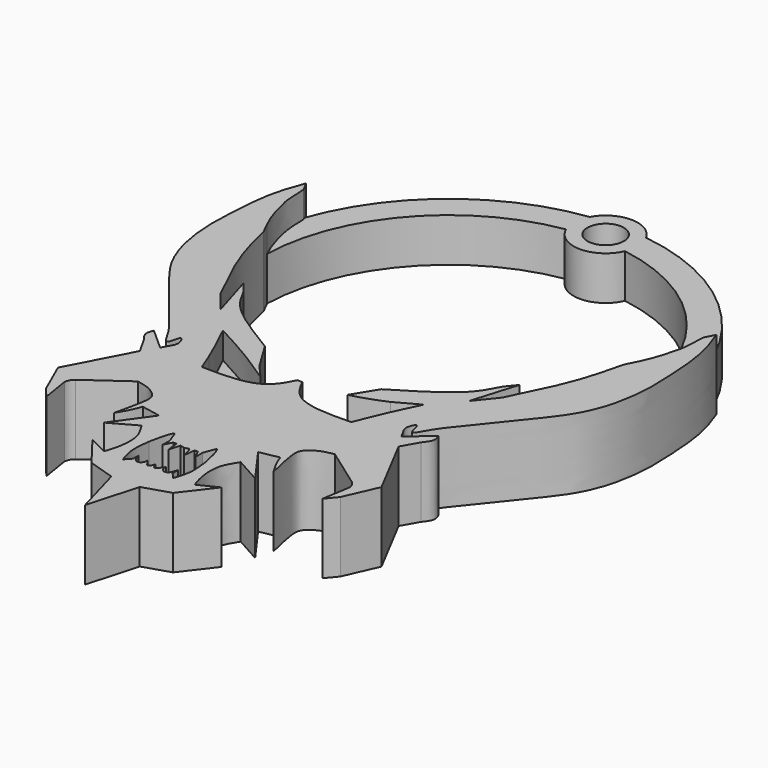
from build123d import *

# Parameters (mm, degrees)
F1_DEPTH = 6.096
F0_R     = 1.5875
F2_DEPTH = 3.81


# Not quite as in the source:
# - a feature names something its author has since deleted; it is built from what else it names


with BuildPart() as f1:
    # F0 (on Top) → F1 (new body)
    with BuildSketch(Plane.XY):
        with BuildLine():
            add(Edge.make_bspline(
                [(0.5293725099, -15.6763419509), (0.5292411185, -15.0751519368), (0.5291231168, -14.1058757461), (-0.304833504, -14.3066064417), (-0.702635768, -15.0022322051), (-0.8362339781, -15.6491980957), (-0.9058115984, -15.9958619624)],
                knots=[0, 0, 0, 0, 0.3108352553, 0.5010759779, 0.7328053585, 1, 1, 1, 1], degree=3))
            Line((-0.9058115984, -15.9958619624), (-0.9058115984, -17.2402724717))
            Line((-0.9058115984, -17.2402724717), (-0.9058115984, -20.226017161))
            Line((-0.9058115984, -20.226017161), (-0.4975165666, -20.1146639884))
            Line((-0.4975165666, -20.1146639884), (-0.2333296888, -21.083349362))
            Line((-0.2333296888, -21.083349362), (-0.120106708, -20.0769230723))
            Line((-0.120106708, -20.0769230723), (0.1692407805, -20.0769230723))
            Line((0.1692407805, -20.0769230723), (0.5214897956, -20.7814220339))
            Line((0.5214897956, -20.7814220339), (0.5214897956, -20.0140215456))
            Line((0.5214897956, -20.0140215456), (0.9240602649, -18.9321134239))
            add(Edge.make_bspline(
                [(1.5430712647, -20.99862881), (1.4140985421, -20.3755580817), (1.2139097457, -19.4084405646), (1.0001161662, -19.0571006756), (0.9240602649, -18.9321134239)],
                knots=[0, 0, 0, 0, 0.6442554471, 1, 1, 1, 1], degree=3))
            add(Edge.make_bspline(
                [(1.5430712647, -20.99862881), (1.5891426732, -21.3454236442), (1.6801064412, -22.0301382187), (1.6564477656, -23.027052549), (1.4157694303, -23.7757681603), (1.2894679367, -24.1686739028)],
                knots=[0, 0, 0, 0, 0.3278252251, 0.6472608224, 1, 1, 1, 1], degree=3))
            Line((1.2894679367, -24.1686739028), (0.8139614056, -23.6456152052))
            Line((0.8139614056, -23.6456152052), (0.8139614056, -23.0591576546))
            Line((0.8139614056, -23.0591576546), (0.6237587932, -23.5980655998))
            add(Edge.make_bspline(
                [(0.6237587932, -23.5980655998), (0.5203329412, -23.7070830693), (0.3117783718, -23.9269129374), (-0.1343922109, -23.6183458648), (-0.1149094653, -23.3495364146), (-0.1053512988, -23.2176594436)],
                knots=[0, 0, 0, 0, 0.3338450489, 0.6731867236, 1, 1, 1, 1], degree=3))
            add(Edge.make_bspline(
                [(-0.1053512988, -23.2176594436), (-0.1910648023, -23.3432038696), (-0.3485399431, -23.5738574464), (-0.6633676878, -23.9588387788), (-0.8187055947, -23.5684484666), (-0.9058115984, -23.3495364146)],
                knots=[0, 0, 0, 0, 0.3441103437, 0.6322087254, 1, 1, 1, 1], degree=3))
            Line((-0.9058115984, -23.3495364146), (-0.9058115984, -31.032309746))
            Line((-0.9058115984, -31.032309746), (0.3292436286, -26.6169421375))
            Line((0.3292436286, -26.6169421375), (2.6450775604, -25.8826520294))
            Line((2.6450775604, -25.8826520294), (4.7067347023, -23.1996756047))
            Line((4.7067347023, -23.1996756047), (3.0404640402, -24.01868999))
            add(Edge.make_bspline(
                [(3.4076086286, -19.4717478007), (3.0937385558, -19.9567840389), (2.4453216005, -20.9588092337), (2.6790373281, -23.0215383373), (2.9334509144, -23.7234480732), (3.0404640402, -24.01868999)],
                knots=[0, 0, 0, 0, 0.352149071, 0.7274966562, 1, 1, 1, 1], degree=3))
            Line((3.4076086286, -19.4717478007), (5.6746407577, -20.7343993974))
            Line((5.6746407577, -20.7343993974), (3.4076086286, -17.5788570195))
            Line((3.4076086286, -17.5788570195), (5.0825377966, -17.2539744526))
            add(Edge.make_bspline(
                [(5.0825377966, -17.2539744526), (4.8011213396, -16.399087297), (4.561581244, -14.6768120309), (3.8789077119, -13.3473311872), (2.9929043757, -14.0969088604), (2.5971549398, -15.3576013762), (2.3466445546, -16.1556228995)],
                knots=[0.2245927854, 0.2245927854, 0.2245927854, 0.2245927854, 0.4782852707, 0.6388064134, 0.7713635541, 1, 1, 1, 1], degree=3))
            add(Edge.make_bspline(
                [(2.3466445546, -16.1556228995), (2.3842676065, -15.6562172431), (2.446566596, -14.829264983), (2.0863685782, -14.1048130028), (1.1405428731, -14.5139735511), (0.7504573644, -15.2558666398), (0.5293725099, -15.6763419509)],
                knots=[0, 0, 0, 0, 0.293818077, 0.4865253721, 0.7089831309, 1, 1, 1, 1], degree=3))
        make_face()
        with BuildLine():
            add(Edge.make_bspline(
                [(-2.3409957066, -15.6763419509), (-2.3408643153, -15.0751519368), (-2.3407463136, -14.1058757461), (-1.5067896928, -14.3066064417), (-1.1089874287, -15.0022322051), (-0.9753892187, -15.6491980957), (-0.9058115984, -15.9958619624)],
                knots=[0, 0, 0, 0, 0.3108352553, 0.5010759779, 0.7328053585, 1, 1, 1, 1], degree=3))
            Line((-0.9058115984, -15.9958619624), (-0.9058115984, -10.0475378801))
            ThreePointArc((-0.9058115984, -10.0475378801), (-2.1470576627, -10.0060667495), (-3.3827675581, -9.8818383259))
            add(Edge.make_bspline(
                [(-7.4073243886, -10.1740490645), (-6.8075722055, -10.1898428856), (-5.6994728773, -10.2190234756), (-4.0527664378, -10.086462301), (-3.3827675581, -9.8818383259)],
                knots=[0, 0, 0, 0, 0.2907722774, 0.5372294996, 0.5372294996, 0.5372294996, 0.5372294996], degree=3))
            add(Edge.make_bspline(
                [(-8.0257326858, -8.6305521925), (-7.8097104935, -9.1525428167), (-7.6085174411, -9.6632959406), (-7.4073243886, -10.1740490645)],
                knots=[0.6828872742, 0.6828872742, 0.6828872742, 0.6828872742, 1, 1, 1, 1], degree=3))
            ThreePointArc((-8.0257326858, -8.6305521925), (-17.8922818311, 0.9803936451), (-18.4399173864, 14.7433572514))
            Line((-18.4399173864, 14.7433572514), (-18.763165921, 15.3649877757))
            add(Edge.make_bspline(
                [(-18.763165921, 15.3649877757), (-19.0883395817, 14.5086239338), (-19.7992570018, 12.636390561), (-20.0614592208, 8.5203671128), (-20.1450147574, 5.8595589947), (-19.6738988858, 2.8012720369), (-18.6296468166, 0.3216380832), (-17.0091341275, -1.7743617945), (-15.3450751303, -3.7604958896), (-13.6655248013, -5.9244622505), (-12.3083012645, -7.5657887279), (-11.4854032906, -9.3943366521), (-11.2878987157, -7.2532302498), (-10.7636393615, -8.3629400774), (-10.8566466443, -8.6570845714), (-10.8958482742, -8.7963175029)],
                knots=[0, 0, 0, 0, 0.0909432234, 0.1983591023, 0.2866981591, 0.3790334905, 0.4664436369, 0.5525333062, 0.6387369107, 0.7267051925, 0.8096970964, 0.865554309, 0.9200718235, 0.9623434622, 1, 1, 1, 1], degree=3))
            Line((-10.8958482742, -8.7963175029), (-11.4042023197, -9.7282994539))
            Line((-11.4042023197, -9.7282994539), (-13.2964076474, -8.0337869003))
            add(Edge.make_bspline(
                [(-13.2964076474, -8.0337869003), (-13.3911344335, -8.2566997732), (-13.5964633769, -8.7398837438), (-13.1995487174, -9.2537872923), (-12.9857473075, -9.5306057483)],
                knots=[0, 0, 0, 0, 0.4613416139, 1, 1, 1, 1], degree=3))
            Line((-12.9857473075, -9.5306057483), (-12.1667329222, -10.9709417447))
            Line((-12.1667329222, -10.9709417447), (-14.9909211323, -16.3651406765))
            Line((-14.9909211323, -16.3651406765), (-13.7200364843, -19.2458126694))
            Line((-13.7200364843, -19.2458126694), (-12.9292635247, -20.2060360461))
            Line((-12.9292635247, -20.2060360461), (-13.3246500045, -17.7489928901))
            add(Edge.make_bspline(
                [(-13.3246500045, -17.7489928901), (-13.3045380935, -17.4936130643), (-13.1847178563, -17.21403189), (-12.9292635247, -17.0147046447)],
                knots=[0, 0, 0, 0, 0.8339722392, 0.8339722392, 0.8339722392, 0.8339722392], degree=3))
            Line((-12.9292635247, -17.0147046447), (-9.4837546349, -14.5576605573))
            add(Edge.make_bspline(
                [(-9.4837546349, -14.5576605573), (-9.1155322754, -14.6255809567), (-8.3698134561, -14.7631324083), (-7.2411030981, -15.5377610794), (-7.2707455103, -16.6588016712), (-7.6292823128, -18.2311499304), (-7.8527219594, -19.2110352218)],
                knots=[0, 0, 0, 0, 0.2233158358, 0.4522561359, 0.6586467707, 1, 1, 1, 1], degree=3))
            add(Edge.make_bspline(
                [(-7.8527219594, -19.2110352218), (-7.4980098211, -18.6109186621), (-7.1432976829, -18.0108021025), (-6.8941609934, -17.2539744526)],
                knots=[0, 0, 0, 0, 0.2245927854, 0.2245927854, 0.2245927854, 0.2245927854], degree=3))
            add(Edge.make_bspline(
                [(-6.8941609934, -17.2539744526), (-6.6127445363, -16.399087297), (-6.3732044408, -14.6768120309), (-5.6905309087, -13.3473311872), (-4.8045275725, -14.0969088604), (-4.4087781365, -15.3576013762), (-4.1582677513, -16.1556228995)],
                knots=[0.2245927854, 0.2245927854, 0.2245927854, 0.2245927854, 0.4782852707, 0.6388064134, 0.7713635541, 1, 1, 1, 1], degree=3))
            add(Edge.make_bspline(
                [(-4.1582677513, -16.1556228995), (-4.1958908032, -15.6562172431), (-4.2581897928, -14.829264983), (-3.897991775, -14.1048130028), (-2.9521660698, -14.5139735511), (-2.5620805612, -15.2558666398), (-2.3409957066, -15.6763419509)],
                knots=[0, 0, 0, 0, 0.293818077, 0.4865253721, 0.7089831309, 1, 1, 1, 1], degree=3))
        make_face()
        with BuildLine():
            Line((-0.9058115984, -17.2402724717), (-0.9058115984, -15.9958619624))
            add(Edge.make_bspline(
                [(-2.3409957066, -15.6763419509), (-2.3408643153, -15.0751519368), (-2.3407463136, -14.1058757461), (-1.5067896928, -14.3066064417), (-1.1089874287, -15.0022322051), (-0.9753892187, -15.6491980957), (-0.9058115984, -15.9958619624)],
                knots=[0, 0, 0, 0, 0.3108352553, 0.5010759779, 0.7328053585, 1, 1, 1, 1], degree=3))
            add(Edge.make_bspline(
                [(-4.1582677513, -16.1556228995), (-4.1958908032, -15.6562172431), (-4.2581897928, -14.829264983), (-3.897991775, -14.1048130028), (-2.9521660698, -14.5139735511), (-2.5620805612, -15.2558666398), (-2.3409957066, -15.6763419509)],
                knots=[0, 0, 0, 0, 0.293818077, 0.4865253721, 0.7089831309, 1, 1, 1, 1], degree=3))
            add(Edge.make_bspline(
                [(-6.8941609934, -17.2539744526), (-6.6127445363, -16.399087297), (-6.3732044408, -14.6768120309), (-5.6905309087, -13.3473311872), (-4.8045275725, -14.0969088604), (-4.4087781365, -15.3576013762), (-4.1582677513, -16.1556228995)],
                knots=[0.2245927854, 0.2245927854, 0.2245927854, 0.2245927854, 0.4782852707, 0.6388064134, 0.7713635541, 1, 1, 1, 1], degree=3))
            Line((-6.8941609934, -17.2539744526), (-5.2192318253, -17.5788570195))
            Line((-5.2192318253, -17.5788570195), (-7.4862639545, -20.7343993974))
            Line((-7.4862639545, -20.7343993974), (-5.2192318253, -19.4717478007))
            add(Edge.make_bspline(
                [(-5.2192318253, -19.4717478007), (-4.9053617526, -19.9567840389), (-4.2569447973, -20.9588092337), (-4.4906605248, -23.0215383373), (-4.7450741111, -23.7234480732), (-4.8520872369, -24.01868999)],
                knots=[0, 0, 0, 0, 0.352149071, 0.7274966562, 1, 1, 1, 1], degree=3))
            Line((-4.8520872369, -24.01868999), (-6.518357899, -23.1996756047))
            Line((-6.518357899, -23.1996756047), (-4.4567007571, -25.8826520294))
            Line((-4.4567007571, -25.8826520294), (-2.1408668254, -26.6169421375))
            Line((-2.1408668254, -26.6169421375), (-0.9058115984, -31.032309746))
            Line((-0.9058115984, -31.032309746), (-0.9058115984, -23.3495364146))
            add(Edge.make_bspline(
                [(-1.706271898, -23.2176594436), (-1.6205583944, -23.3432038696), (-1.4630832536, -23.5738574464), (-1.148255509, -23.9588387788), (-0.992917602, -23.5684484666), (-0.9058115984, -23.3495364146)],
                knots=[0, 0, 0, 0, 0.3441103437, 0.6322087254, 1, 1, 1, 1], degree=3))
            add(Edge.make_bspline(
                [(-2.4353819899, -23.5980655998), (-2.331956138, -23.7070830693), (-2.1234015686, -23.9269129374), (-1.6772309858, -23.6183458648), (-1.6967137315, -23.3495364146), (-1.706271898, -23.2176594436)],
                knots=[0, 0, 0, 0, 0.3338450489, 0.6731867236, 1, 1, 1, 1], degree=3))
            Line((-2.4353819899, -23.5980655998), (-2.6255846024, -23.0591576546))
            Line((-2.6255846024, -23.0591576546), (-2.6255846024, -23.6456152052))
            Line((-2.6255846024, -23.6456152052), (-3.1010911334, -24.1686739028))
            add(Edge.make_bspline(
                [(-3.3546944614, -20.99862881), (-3.4007658699, -21.3454236442), (-3.491729638, -22.0301382187), (-3.4680709624, -23.027052549), (-3.2273926271, -23.7757681603), (-3.1010911334, -24.1686739028)],
                knots=[0, 0, 0, 0, 0.3278252251, 0.6472608224, 1, 1, 1, 1], degree=3))
            add(Edge.make_bspline(
                [(-3.3546944614, -20.99862881), (-3.2257217389, -20.3755580817), (-3.0255329424, -19.4084405646), (-2.811739363, -19.0571006756), (-2.7356834617, -18.9321134239)],
                knots=[0, 0, 0, 0, 0.6442554471, 1, 1, 1, 1], degree=3))
            Line((-2.7356834617, -18.9321134239), (-2.3331129923, -20.0140215456))
            Line((-2.3331129923, -20.0140215456), (-2.3331129923, -20.7814220339))
            Line((-2.3331129923, -20.7814220339), (-1.9808639772, -20.0769230723))
            Line((-1.9808639772, -20.0769230723), (-1.6915164888, -20.0769230723))
            Line((-1.6915164888, -20.0769230723), (-1.5782935079, -21.083349362))
            Line((-1.5782935079, -21.083349362), (-1.3141066302, -20.1146639884))
            Line((-1.3141066302, -20.1146639884), (-0.9058115984, -20.226017161))
            Line((-0.9058115984, -20.226017161), (-0.9058115984, -17.2402724717))
        make_face()
        with BuildLine():
            Line((-0.9058115984, -10.0475378801), (-0.9058115984, -15.9958619624))
            add(Edge.make_bspline(
                [(0.5293725099, -15.6763419509), (0.5292411185, -15.0751519368), (0.5291231168, -14.1058757461), (-0.304833504, -14.3066064417), (-0.702635768, -15.0022322051), (-0.8362339781, -15.6491980957), (-0.9058115984, -15.9958619624)],
                knots=[0, 0, 0, 0, 0.3108352553, 0.5010759779, 0.7328053585, 1, 1, 1, 1], degree=3))
            add(Edge.make_bspline(
                [(2.3466445546, -16.1556228995), (2.3842676065, -15.6562172431), (2.446566596, -14.829264983), (2.0863685782, -14.1048130028), (1.1405428731, -14.5139735511), (0.7504573644, -15.2558666398), (0.5293725099, -15.6763419509)],
                knots=[0, 0, 0, 0, 0.293818077, 0.4865253721, 0.7089831309, 1, 1, 1, 1], degree=3))
            add(Edge.make_bspline(
                [(5.0825377966, -17.2539744526), (4.8011213396, -16.399087297), (4.561581244, -14.6768120309), (3.8789077119, -13.3473311872), (2.9929043757, -14.0969088604), (2.5971549398, -15.3576013762), (2.3466445546, -16.1556228995)],
                knots=[0.2245927854, 0.2245927854, 0.2245927854, 0.2245927854, 0.4782852707, 0.6388064134, 0.7713635541, 1, 1, 1, 1], degree=3))
            add(Edge.make_bspline(
                [(6.0410987626, -19.2110352218), (5.6863866244, -18.6109186621), (5.3316744862, -18.0108021025), (5.0825377966, -17.2539744526)],
                knots=[0, 0, 0, 0, 0.2245927854, 0.2245927854, 0.2245927854, 0.2245927854], degree=3))
            add(Edge.make_bspline(
                [(7.6721314381, -14.5576605573), (7.3039090787, -14.6255809567), (6.5581902593, -14.7631324083), (5.4294799013, -15.5377610794), (5.4591223135, -16.6588016712), (5.8176591161, -18.2311499304), (6.0410987626, -19.2110352218)],
                knots=[0, 0, 0, 0, 0.2233158358, 0.4522561359, 0.6586467707, 1, 1, 1, 1], degree=3))
            Line((7.6721314381, -14.5576605573), (11.117640328, -17.0147046447))
            add(Edge.make_bspline(
                [(11.5130268078, -17.7489928901), (11.4929148968, -17.4936130643), (11.3730946596, -17.21403189), (11.117640328, -17.0147046447)],
                knots=[0, 0, 0, 0, 0.8339722392, 0.8339722392, 0.8339722392, 0.8339722392], degree=3))
            Line((11.5130268078, -17.7489928901), (11.117640328, -20.2060360461))
            Line((11.117640328, -20.2060360461), (11.9084132875, -19.2458126694))
            Line((11.9084132875, -19.2458126694), (13.1792979355, -16.3651406765))
            Line((13.1792979355, -16.3651406765), (10.3551097254, -10.9709417447))
            Line((10.3551097254, -10.9709417447), (11.1741241108, -9.5306057483))
            add(Edge.make_bspline(
                [(11.4847844507, -8.0337869003), (11.5795112368, -8.2566997732), (11.7848401801, -8.7398837438), (11.3879255207, -9.2537872923), (11.1741241108, -9.5306057483)],
                knots=[0, 0, 0, 0, 0.4613416139, 1, 1, 1, 1], degree=3))
            Line((11.4847844507, -8.0337869003), (9.5925791229, -9.7282994539))
            Line((9.5925791229, -9.7282994539), (9.0842250775, -8.7963175029))
            add(Edge.make_bspline(
                [(16.9515427242, 15.3649877757), (17.276716385, 14.5086239338), (17.9876338051, 12.636390561), (18.249836024, 8.5203671128), (18.3333915607, 5.8595589947), (17.862275689, 2.8012720369), (16.8180236199, 0.3216380832), (15.1975109308, -1.7743617945), (13.5334519336, -3.7604958896), (11.8539016046, -5.9244622505), (10.4966780678, -7.5657887279), (9.6737800938, -9.3943366521), (9.4762755189, -7.2532302498), (8.9520161648, -8.3629400774), (9.0450234476, -8.6570845714), (9.0842250775, -8.7963175029)],
                knots=[0, 0, 0, 0, 0.0909432234, 0.1983591023, 0.2866981591, 0.3790334905, 0.4664436369, 0.5525333062, 0.6387369107, 0.7267051925, 0.8096970964, 0.865554309, 0.9200718235, 0.9623434622, 1, 1, 1, 1], degree=3))
            Line((16.9515427242, 15.3649877757), (16.6282941897, 14.7433572514))
            ThreePointArc((16.6282941897, 14.7433572514), (16.0806586343, 0.9803936451), (6.214109489, -8.6305521925))
            add(Edge.make_bspline(
                [(6.214109489, -8.6305521925), (5.9980872968, -9.1525428167), (5.7968942443, -9.6632959406), (5.5957011919, -10.1740490645)],
                knots=[0.6828872742, 0.6828872742, 0.6828872742, 0.6828872742, 1, 1, 1, 1], degree=3))
            add(Edge.make_bspline(
                [(5.5957011919, -10.1740490645), (4.9959490087, -10.1898428856), (3.8878496805, -10.2190234756), (2.241143241, -10.086462301), (1.5711443613, -9.8818383259)],
                knots=[0, 0, 0, 0, 0.2907722774, 0.5372294996, 0.5372294996, 0.5372294996, 0.5372294996], degree=3))
            ThreePointArc((1.5711443613, -9.8818383259), (0.3354344659, -10.0060667495), (-0.9058115984, -10.0475378801))
        make_face()
        with BuildLine():
            ThreePointArc((-3.3827675581, -9.8818383259), (-2.1470576627, -10.0060667495), (-0.9058115984, -10.0475378801))
            Line((-0.9058115984, -10.0475378801), (-0.9058115984, -7.6482766994))
            ThreePointArc((-0.9058115984, -7.6482766994), (-1.0157079575, -7.6479038715), (-1.1255992574, -7.6467854049))
            add(Edge.make_bspline(
                [(-3.3827675581, -9.8818383259), (-3.074878211, -9.7878060164), (-2.0439464299, -9.3453334482), (-1.4853159333, -8.3839003279), (-1.1255992574, -7.6467854049)],
                knots=[0.5372294996, 0.5372294996, 0.5372294996, 0.5372294996, 0.6504857386, 0.9400606426, 0.9400606426, 0.9400606426, 0.9400606426], degree=3))
        make_face()
        with BuildLine():
            Line((-0.9058115984, -7.6482766994), (-0.9058115984, -10.0475378801))
            ThreePointArc((-0.9058115984, -10.0475378801), (0.3354344659, -10.0060667495), (1.5711443613, -9.8818383259))
            add(Edge.make_bspline(
                [(1.5711443613, -9.8818383259), (1.2632550142, -9.7878060164), (0.2323232332, -9.3453334482), (-0.3263072635, -8.3839003279), (-0.6860239394, -7.6467854049)],
                knots=[0.5372294996, 0.5372294996, 0.5372294996, 0.5372294996, 0.6504857386, 0.9400606426, 0.9400606426, 0.9400606426, 0.9400606426], degree=3))
            ThreePointArc((-0.6860239394, -7.6467854049), (-0.7959152393, -7.6479038715), (-0.9058115984, -7.6482766994))
        make_face()
        with BuildLine():
            ThreePointArc((-18.4399173864, 14.7433572514), (-17.8922818311, 0.9803936451), (-8.0257326858, -8.6305521925))
            add(Edge.make_bspline(
                [(-9.649024345, -5.0857467577), (-9.2018465181, -6.0143296372), (-8.6167744293, -7.2292555399), (-8.1353730658, -8.3656199195), (-8.0257326858, -8.6305521925)],
                knots=[0, 0, 0, 0, 0.5219391817, 0.6828872742, 0.6828872742, 0.6828872742, 0.6828872742], degree=3))
            add(Edge.make_bspline(
                [(-3.3968286589, -8.8159106672), (-4.3297126076, -8.1952203913), (-6.2560722042, -6.9135254161), (-8.4945703967, -5.7076495141), (-9.649024345, -5.0857467577)],
                knots=[0, 0, 0, 0, 0.484273004, 1, 1, 1, 1], degree=3))
            Line((-3.3968286589, -8.8159106672), (-4.4557689689, -7.6074535027))
            Line((-4.4557689689, -7.6074535027), (-4.7058596813, -7.1961932321))
            Line((-4.7058596813, -7.1961932321), (-5.9671136551, -5.1221312024))
            add(Edge.make_bspline(
                [(-12.2140059248, 0.3858812852), (-11.8433550049, -0.3271820386), (-11.0389490239, -1.8747092988), (-8.1365297729, -3.8021083616), (-6.6544101224, -4.7039324862), (-5.9671136551, -5.1221312024)],
                knots=[0, 0, 0, 0, 0.3142491652, 0.6819999478, 1, 1, 1, 1], degree=3))
            Line((-12.2140059248, 0.3858812852), (-12.9192993045, 1.2591026025))
            Line((-12.9192993045, 1.2591026025), (-11.7197120562, -2.7457582764))
            Line((-11.7197120562, -2.7457582764), (-13.1711000577, -0.9362358251))
            add(Edge.make_bspline(
                [(-13.1711000577, -0.9362358251), (-13.7429419596, 0.2298490954), (-15.2568416961, 3.2091643903), (-16.0208158195, 5.6008263491), (-16.5893193334, 8.0244466662)],
                knots=[0, 0, 0, 0, 0.4713548549, 1, 1, 1, 1], degree=3))
            add(Edge.make_bspline(
                [(-17.0952569714, 9.041607067), (-16.9341185587, 8.7018864406), (-16.7617189461, 8.3631665534), (-16.5893193334, 8.0244466662)],
                knots=[0.8528354417, 0.8528354417, 0.8528354417, 0.8528354417, 1, 1, 1, 1], degree=3))
            add(Edge.make_bspline(
                [(-18.3265544474, 14.5253520459), (-18.3081715606, 13.8728301779), (-18.2756177744, 12.7172958195), (-18.0204633198, 11.6637036696), (-17.6484482316, 10.2698438195), (-17.2464131515, 9.3602826165), (-17.0952569714, 9.041607067)],
                knots=[0, 0, 0, 0, 0.2597054553, 0.459905777, 0.714787461, 0.8528354417, 0.8528354417, 0.8528354417, 0.8528354417], degree=3))
            Line((-18.3265544474, 14.5253520459), (-18.4399173864, 14.7433572514))
        make_face()
        with BuildLine():
            add(Edge.make_bspline(
                [(7.8374011482, -5.0857467577), (7.3902233214, -6.0143296372), (6.8051512326, -7.2292555399), (6.3237498691, -8.3656199195), (6.214109489, -8.6305521925)],
                knots=[0, 0, 0, 0, 0.5219391817, 0.6828872742, 0.6828872742, 0.6828872742, 0.6828872742], degree=3))
            ThreePointArc((6.214109489, -8.6305521925), (16.0806586343, 0.9803936451), (16.6282941897, 14.7433572514))
            Line((16.6282941897, 14.7433572514), (16.5149312507, 14.5253520459))
            add(Edge.make_bspline(
                [(16.5149312507, 14.5253520459), (16.4965483638, 13.8728301779), (16.4639945776, 12.7172958195), (16.208840123, 11.6637036696), (15.8368250348, 10.2698438195), (15.4347899547, 9.3602826165), (15.2836337746, 9.041607067)],
                knots=[0, 0, 0, 0, 0.2597054553, 0.459905777, 0.714787461, 0.8528354417, 0.8528354417, 0.8528354417, 0.8528354417], degree=3))
            add(Edge.make_bspline(
                [(15.2836337746, 9.041607067), (15.1224953619, 8.7018864406), (14.9500957493, 8.3631665534), (14.7776961367, 8.0244466662)],
                knots=[0.8528354417, 0.8528354417, 0.8528354417, 0.8528354417, 1, 1, 1, 1], degree=3))
            add(Edge.make_bspline(
                [(11.3594768609, -0.9362358251), (11.9313187629, 0.2298490954), (13.4452184993, 3.2091643903), (14.2091926227, 5.6008263491), (14.7776961367, 8.0244466662)],
                knots=[0, 0, 0, 0, 0.4713548549, 1, 1, 1, 1], degree=3))
            Line((11.3594768609, -0.9362358251), (9.9080888595, -2.7457582764))
            Line((9.9080888595, -2.7457582764), (11.1076761077, 1.2591026025))
            Line((11.1076761077, 1.2591026025), (10.402382728, 0.3858812852))
            add(Edge.make_bspline(
                [(10.402382728, 0.3858812852), (10.0317318081, -0.3271820386), (9.2273258271, -1.8747092988), (6.3249065761, -3.8021083616), (4.8427869256, -4.7039324862), (4.1554904583, -5.1221312024)],
                knots=[0, 0, 0, 0, 0.3142491652, 0.6819999478, 1, 1, 1, 1], degree=3))
            Line((4.1554904583, -5.1221312024), (2.8942364845, -7.1961932321))
            ThreePointArc((2.8942364845, -7.1961932321), (4.3806415548, -6.7612776776), (5.8187132559, -6.1863852052))
            add(Edge.make_bspline(
                [(5.8187132559, -6.1863852052), (6.4803724044, -5.8167762783), (7.1588867763, -5.451261518), (7.8374011482, -5.0857467577)],
                knots=[0.6968885772, 0.6968885772, 0.6968885772, 0.6968885772, 1, 1, 1, 1], degree=3))
        make_face()
    extrude(amount=F1_DEPTH)

    # F0 (on Top) → F2 (join)
    with BuildSketch(Plane.XY):
        with BuildLine():
            ThreePointArc((-3.3541433936, 26.983005386), (-12.6223255661, 22.9896650878), (-18.4399173864, 14.7433572514))
            Line((-18.4399173864, 14.7433572514), (-18.3265544474, 14.5253520459))
            add(Edge.make_bspline(
                [(-18.3265544474, 14.5253520459), (-18.3081715606, 13.8728301779), (-18.2756177744, 12.7172958195), (-18.0204633198, 11.6637036696), (-17.6484482316, 10.2698438195), (-17.2464131515, 9.3602826165), (-17.0952569714, 9.041607067)],
                knots=[0, 0, 0, 0, 0.2597054553, 0.459905777, 0.714787461, 0.8528354417, 0.8528354417, 0.8528354417, 0.8528354417], degree=3))
            ThreePointArc((-17.0952569714, 9.041607067), (-13.0710109293, 19.2420830109), (-3.4708360315, 24.5412251699))
            ThreePointArc((-3.4708360315, 24.5412251699), (-0.9058115984, 22.8509482565), (1.6592128348, 24.5412251699))
            ThreePointArc((1.6592128348, 24.5412251699), (11.2593877326, 19.2420830109), (15.2836337746, 9.041607067))
            add(Edge.make_bspline(
                [(16.5149312507, 14.5253520459), (16.4965483638, 13.8728301779), (16.4639945776, 12.7172958195), (16.208840123, 11.6637036696), (15.8368250348, 10.2698438195), (15.4347899547, 9.3602826165), (15.2836337746, 9.041607067)],
                knots=[0, 0, 0, 0, 0.2597054553, 0.459905777, 0.714787461, 0.8528354417, 0.8528354417, 0.8528354417, 0.8528354417], degree=3))
            Line((16.5149312507, 14.5253520459), (16.6282941897, 14.7433572514))
            ThreePointArc((16.6282941897, 14.7433572514), (10.8107023694, 22.9896650878), (1.5425201968, 26.983005386))
            ThreePointArc((1.5425201968, 26.983005386), (-0.9058115984, 28.4336940845), (-3.3541433936, 26.983005386))
        make_face()
        with Locations((-0.9058115984, 25.6423211705)):
            Circle(F0_R, mode=Mode.SUBTRACT)
        with BuildLine():
            ThreePointArc((-8.0257326858, -8.6305521925), (-5.744865381, -9.406900383), (-3.3827675581, -9.8818383259))
            add(Edge.make_bspline(
                [(-3.3827675581, -9.8818383259), (-3.074878211, -9.7878060164), (-2.0439464299, -9.3453334482), (-1.4853159333, -8.3839003279), (-1.1255992574, -7.6467854049)],
                knots=[0.5372294996, 0.5372294996, 0.5372294996, 0.5372294996, 0.6504857386, 0.9400606426, 0.9400606426, 0.9400606426, 0.9400606426], degree=3))
            ThreePointArc((-1.1255992574, -7.6467854049), (-2.9283170185, -7.5215059343), (-4.7058596813, -7.1961932321))
            Line((-4.7058596813, -7.1961932321), (-4.4557689689, -7.6074535027))
            Line((-4.4557689689, -7.6074535027), (-3.3968286589, -8.8159106672))
            add(Edge.make_bspline(
                [(-3.3968286589, -8.8159106672), (-4.3297126076, -8.1952203913), (-6.2560722042, -6.9135254161), (-8.4945703967, -5.7076495141), (-9.649024345, -5.0857467577)],
                knots=[0, 0, 0, 0, 0.484273004, 1, 1, 1, 1], degree=3))
            add(Edge.make_bspline(
                [(-9.649024345, -5.0857467577), (-9.2018465181, -6.0143296372), (-8.6167744293, -7.2292555399), (-8.1353730658, -8.3656199195), (-8.0257326858, -8.6305521925)],
                knots=[0, 0, 0, 0, 0.5219391817, 0.6828872742, 0.6828872742, 0.6828872742, 0.6828872742], degree=3))
        make_face()
        with BuildLine():
            add(Edge.make_bspline(
                [(1.5711443613, -9.8818383259), (1.2632550142, -9.7878060164), (0.2323232332, -9.3453334482), (-0.3263072635, -8.3839003279), (-0.6860239394, -7.6467854049)],
                knots=[0.5372294996, 0.5372294996, 0.5372294996, 0.5372294996, 0.6504857386, 0.9400606426, 0.9400606426, 0.9400606426, 0.9400606426], degree=3))
            ThreePointArc((1.5711443613, -9.8818383259), (3.9332421843, -9.406900383), (6.214109489, -8.6305521925))
            add(Edge.make_bspline(
                [(7.8374011482, -5.0857467577), (7.3902233214, -6.0143296372), (6.8051512326, -7.2292555399), (6.3237498691, -8.3656199195), (6.214109489, -8.6305521925)],
                knots=[0, 0, 0, 0, 0.5219391817, 0.6828872742, 0.6828872742, 0.6828872742, 0.6828872742], degree=3))
            ThreePointArc((7.8374011482, -5.0857467577), (6.8476120242, -5.6719316035), (5.8187132559, -6.1863852052))
            add(Edge.make_bspline(
                [(1.5852054621, -8.8159106672), (2.5180894108, -8.1952203913), (3.8605474094, -7.3020218036), (5.3545966685, -6.4456450284), (5.8187132559, -6.1863852052)],
                knots=[0, 0, 0, 0, 0.484273004, 0.6968885772, 0.6968885772, 0.6968885772, 0.6968885772], degree=3))
            Line((1.5852054621, -8.8159106672), (2.6441457722, -7.6074535027))
            Line((2.6441457722, -7.6074535027), (2.8942364845, -7.1961932321))
            ThreePointArc((2.8942364845, -7.1961932321), (1.1166938218, -7.5215059343), (-0.6860239394, -7.6467854049))
        make_face()
        with BuildLine():
            ThreePointArc((-18.4399173864, 14.7433572514), (-17.8922818311, 0.9803936451), (-8.0257326858, -8.6305521925))
            add(Edge.make_bspline(
                [(-9.649024345, -5.0857467577), (-9.2018465181, -6.0143296372), (-8.6167744293, -7.2292555399), (-8.1353730658, -8.3656199195), (-8.0257326858, -8.6305521925)],
                knots=[0, 0, 0, 0, 0.5219391817, 0.6828872742, 0.6828872742, 0.6828872742, 0.6828872742], degree=3))
            add(Edge.make_bspline(
                [(-3.3968286589, -8.8159106672), (-4.3297126076, -8.1952203913), (-6.2560722042, -6.9135254161), (-8.4945703967, -5.7076495141), (-9.649024345, -5.0857467577)],
                knots=[0, 0, 0, 0, 0.484273004, 1, 1, 1, 1], degree=3))
            Line((-3.3968286589, -8.8159106672), (-4.4557689689, -7.6074535027))
            Line((-4.4557689689, -7.6074535027), (-4.7058596813, -7.1961932321))
            Line((-4.7058596813, -7.1961932321), (-5.9671136551, -5.1221312024))
            add(Edge.make_bspline(
                [(-12.2140059248, 0.3858812852), (-11.8433550049, -0.3271820386), (-11.0389490239, -1.8747092988), (-8.1365297729, -3.8021083616), (-6.6544101224, -4.7039324862), (-5.9671136551, -5.1221312024)],
                knots=[0, 0, 0, 0, 0.3142491652, 0.6819999478, 1, 1, 1, 1], degree=3))
            Line((-12.2140059248, 0.3858812852), (-12.9192993045, 1.2591026025))
            Line((-12.9192993045, 1.2591026025), (-11.7197120562, -2.7457582764))
            Line((-11.7197120562, -2.7457582764), (-13.1711000577, -0.9362358251))
            add(Edge.make_bspline(
                [(-13.1711000577, -0.9362358251), (-13.7429419596, 0.2298490954), (-15.2568416961, 3.2091643903), (-16.0208158195, 5.6008263491), (-16.5893193334, 8.0244466662)],
                knots=[0, 0, 0, 0, 0.4713548549, 1, 1, 1, 1], degree=3))
            add(Edge.make_bspline(
                [(-17.0952569714, 9.041607067), (-16.9341185587, 8.7018864406), (-16.7617189461, 8.3631665534), (-16.5893193334, 8.0244466662)],
                knots=[0.8528354417, 0.8528354417, 0.8528354417, 0.8528354417, 1, 1, 1, 1], degree=3))
            add(Edge.make_bspline(
                [(-18.3265544474, 14.5253520459), (-18.3081715606, 13.8728301779), (-18.2756177744, 12.7172958195), (-18.0204633198, 11.6637036696), (-17.6484482316, 10.2698438195), (-17.2464131515, 9.3602826165), (-17.0952569714, 9.041607067)],
                knots=[0, 0, 0, 0, 0.2597054553, 0.459905777, 0.714787461, 0.8528354417, 0.8528354417, 0.8528354417, 0.8528354417], degree=3))
            Line((-18.3265544474, 14.5253520459), (-18.4399173864, 14.7433572514))
        make_face()
        with BuildLine():
            ThreePointArc((5.8187132559, -6.1863852052), (4.3806415548, -6.7612776776), (2.8942364845, -7.1961932321))
            Line((2.8942364845, -7.1961932321), (2.6441457722, -7.6074535027))
            Line((2.6441457722, -7.6074535027), (1.5852054621, -8.8159106672))
            add(Edge.make_bspline(
                [(1.5852054621, -8.8159106672), (2.5180894108, -8.1952203913), (3.8605474094, -7.3020218036), (5.3545966685, -6.4456450284), (5.8187132559, -6.1863852052)],
                knots=[0, 0, 0, 0, 0.484273004, 0.6968885772, 0.6968885772, 0.6968885772, 0.6968885772], degree=3))
        make_face()
    extrude(amount=F2_DEPTH)


solid = f1.part
